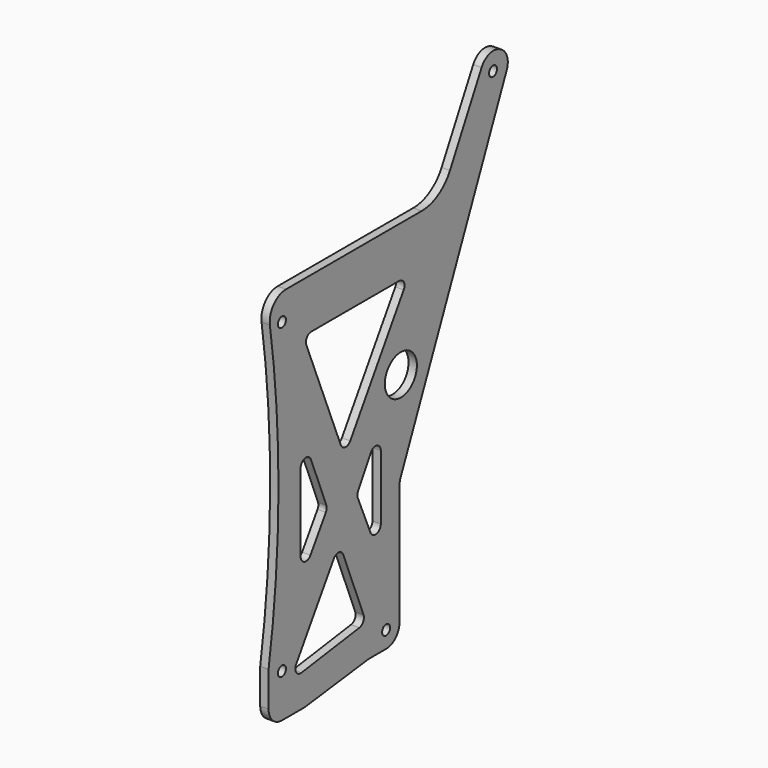
from build123d import *

# Parameters (mm, degrees)
F0_R     = 1.5
F0_R_2   = 6
F1_DEPTH = 1.25


# Not quite as in the source:
# - ends of sketch curves that miss each other by under 0.0002 mm in the source are joined


with BuildPart() as f1:
    # F0 (on Right) → F1 (new body, symmetric)
    with BuildSketch(Plane.YZ):
        with BuildLine():
            ThreePointArc((-44.2615727709, 33.8276430339), (-41.0580126337, -11.4414374496), (-44.7615726272, -56.6723570594))
            Line((-44.7615726272, -56.6723570594), (-44.761573, -67.172357))
            ThreePointArc((-44.761573, -67.172357), (-43.2971069059, -70.7078909059), (-39.761573, -72.172357))
            Line((-39.761573, -72.172357), (-31.572862, -72.172357))
            ThreePointArc((-31.572862, -72.172357), (-31.2621746065, -72.1626949989), (-30.9526879578, -72.1337463374))
            Line((-30.9526879578, -72.1337463374), (-7.570458, -69.210968))
            ThreePointArc((-7.570458, -69.210968), (-7.2609713935, -69.1820190011), (-6.950284, -69.172357))
            Line((-6.950284, -69.172357), (-0.761573, -69.172357))
            ThreePointArc((-0.761573, -69.172357), (2.7739609059, -67.7078909059), (4.238427, -64.172357))
            Line((4.238427, -64.172357), (4.238427, -28.200354))
            ThreePointArc((4.238427, -28.200354), (4.340868282, -27.1934187471), (4.6439944414, -26.2277441895))
            Line((4.6439944414, -26.2277441895), (44.34607, 64.980308))
            ThreePointArc((44.34607, 64.980308), (44.4613498885, 68.6823868), (41.9976409775, 71.448035955))
            Line((41.9976409775, 71.448035955), (41.604729, 71.644492))
            ThreePointArc((41.604729, 71.644492), (37.8444305073, 71.9343641274), (34.9513503203, 69.5148688301))
            Line((34.9513503203, 69.5148688301), (23.120683, 47.205611))
            ThreePointArc((23.120683, 47.205611), (18.7052359642, 42.5450269916), (12.519138, 40.827643))
            Line((12.519138, 40.827643), (-38.220653, 40.827643))
            ThreePointArc((-38.220653, 40.827643), (-42.8437667533, 38.710714686), (-44.2615727709, 33.8276430339))
        make_face()
        with Locations((-39.761573, -59.172357)):
            Circle(F0_R, mode=Mode.SUBTRACT)
        with Locations((-0.761573, -64.172357)):
            Circle(F0_R, mode=Mode.SUBTRACT)
        with BuildLine():
            ThreePointArc((-9.2090828941, -56.8035819576), (-9.3358141293, -58.5495251427), (-10.7880590013, -59.5269519905))
            Line((-10.7880590013, -59.5269519905), (-32.462939, -62.56904))
            ThreePointArc((-32.462939, -62.56904), (-34.4234257272, -61.6697294934), (-34.4270410919, -59.5128209413))
            Line((-34.4270410919, -59.5128209413), (-20.357382, -37.45768))
            ThreePointArc((-20.357382, -37.45768), (-18.4841932611, -36.5420784276), (-16.8143035493, -37.7905298197))
            Line((-16.8143035493, -37.7905298197), (-9.2090828941, -56.8035819576))
        make_face(mode=Mode.SUBTRACT)
        with BuildLine():
            Line((-23.321557, -24.040332), (-29.08098, -32.967437))
            ThreePointArc((-29.08098, -32.967437), (-31.3267335557, -33.8016713068), (-32.761573, -31.883184))
            Line((-32.761573, -31.883184), (-32.761573, -8.557522))
            ThreePointArc((-32.761573, -8.557522), (-31.139788407, -6.5936092968), (-28.9046198941, -7.8147399576))
            Line((-28.9046198941, -7.8147399576), (-23.145197, -22.213297))
            ThreePointArc((-23.145197, -22.213297), (-23.0114029888, -23.1482412686), (-23.321557, -24.040332))
        make_face(mode=Mode.SUBTRACT)
        with BuildLine():
            ThreePointArc((-11.3658482669, -25.0957141144), (-11.5238882865, -24.1867752684), (-11.2571359352, -23.3036050376))
            Line((-11.2571359352, -23.3036050376), (-6.491151, -15.095519))
            ThreePointArc((-6.491151, -15.095519), (-4.2415517843, -14.1685784799), (-2.761573, -16.09979))
            Line((-2.761573, -16.09979), (-2.761573, -35.428508))
            ThreePointArc((-2.761573, -35.428508), (-4.3594410625, -37.387663406), (-6.5998629049, -36.2163469592))
            Line((-6.5998629049, -36.2163469592), (-11.3658482669, -25.0957141144))
        make_face(mode=Mode.SUBTRACT)
        with Locations((-39.761573, 32.827643)):
            Circle(F0_R, mode=Mode.SUBTRACT)
        with BuildLine():
            Line((5.800752, 22.759657), (-14.186435, -8.886721))
            ThreePointArc((-14.186435, -8.886721), (-16.0532082809, -9.8109940241), (-17.7292820906, -8.574103037))
            Line((-17.7292820906, -8.574103037), (-30.637673, 23.072275))
            ThreePointArc((-30.637673, 23.072275), (-30.4457341301, 24.9432737467), (-28.785804, 25.827643))
            Line((-28.785804, 25.827643), (4.109774, 25.827643))
            ThreePointArc((4.109774, 25.827643), (5.8613407009, 24.7930517696), (5.800752, 22.759657))
        make_face(mode=Mode.SUBTRACT)
        with Locations((4.738427, 0.827643)):
            Circle(F0_R_2, mode=Mode.SUBTRACT)
        with Locations((39.238427, 66.827643)):
            Circle(F0_R, mode=Mode.SUBTRACT)
    extrude(amount=F1_DEPTH, both=True)


solid = f1.part
